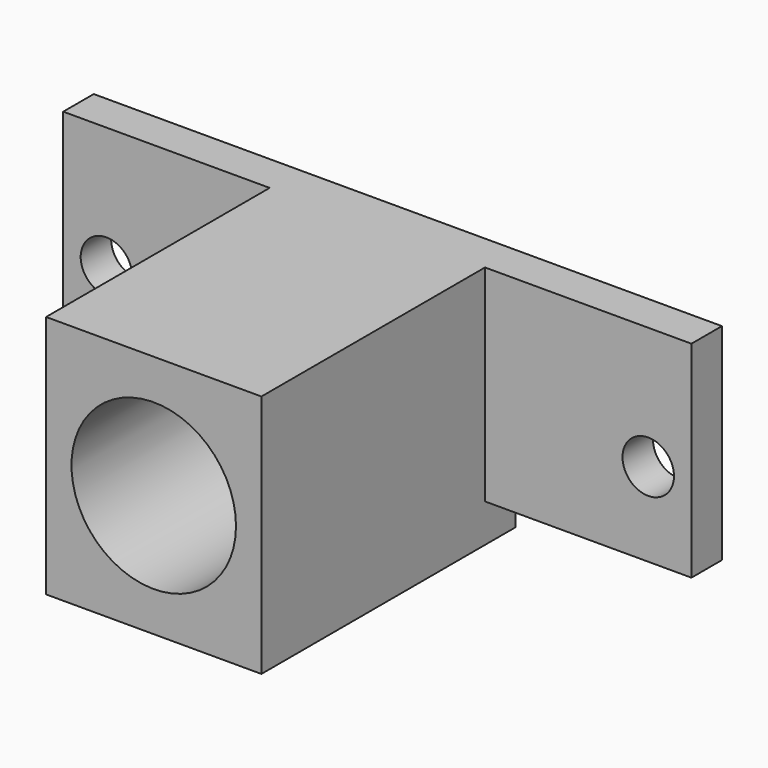
from build123d import *

# Parameters (mm, degrees)
F0_W         = 17.2212
F0_H         = 19.5351538889
F0_R         = 6.5786
F1_DEPTH     = 25.4
F2_R         = 2.0574
F2_W         = 16.51
F2_H         = 16.51
F3_DEPTH     = 3.048
F4_TEXT_SIZE = 2.3282805665
F5_DEPTH     = 22.86
F6_W         = 13.208
F6_H         = 11.43
F7_DEPTH     = 10.16


# Not quite as in the source:
# - a feature names something its author has since deleted; it is built from what else it names
# - Text() gives the source's letters only with a copy of the font that has no kerning and outlines rounded to 1/6400 em; it was checked with that copy


with BuildPart() as f1:
    # F0 (on Front) → F1 (new body)
    with BuildSketch(Plane.XZ):
        with Locations((-32.2175832933, 21.9545621703)):
            Rectangle(F0_W, F0_H)
        with Locations((-32.2175832933, 21.9405852258)):
            Circle(F0_R, mode=Mode.SUBTRACT)
    extrude(amount=F1_DEPTH)

    # F2 (on Front) → F3 (join)
    with BuildSketch(Plane.XZ):
        Polygon((-7.0969832933, 31.7221391147), (-23.6069832933, 31.7221391147), (-23.6069832933, 15.2479470575), (-8.3669832933, 15.2479470575), (-7.0969832933, 15.2479470575), align=None)
        with Locations((-10.5513832933, 21.9405852258)):
            Circle(F2_R, mode=Mode.SUBTRACT)
        with Locations((-49.0831832933, 23.4671391147)):
            Rectangle(F2_W, F2_H)
        with Locations((-53.8837832933, 21.9405852258)):
            Circle(F2_R, mode=Mode.SUBTRACT)
    extrude(amount=F3_DEPTH)

    # F4 (on Front) → F5 (join)
    with BuildSketch(Plane.XZ):
        with Locations((-34.7727015615, 29.5575335622)):
            Text('R.P.U', F4_TEXT_SIZE, font='Open Sans', font_style=FontStyle.BOLD, text_align=(TextAlign.LEFT, TextAlign.BOTTOM))
    extrude(amount=F5_DEPTH)

    # F6 (on Front) → F7 (cut)
    with BuildSketch(Plane.XZ):
        with Locations((-32.0291832501, 22.4511391147)):
            Rectangle(F6_W, F6_H)
    extrude(amount=F7_DEPTH, mode=Mode.SUBTRACT)


solid = f1.part
